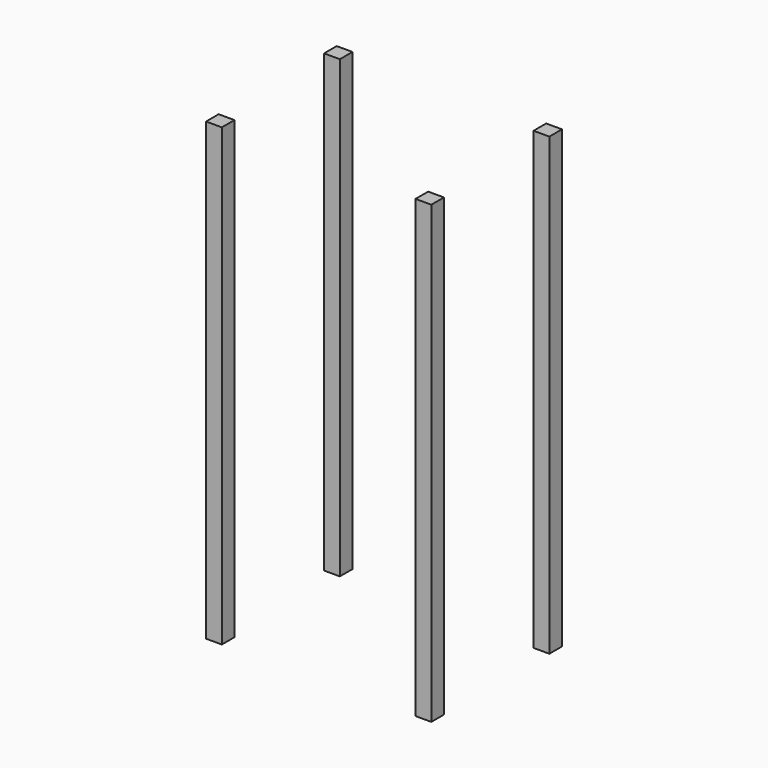
from build123d import *

# Parameters (mm, degrees)
F0_W     = 5.08
F0_H     = 5.08
F1_DEPTH = 146.41856


# Not quite as in the source:
# - the program builds the solid bodies; features that only make, move or delete a surface that nothing else refers to are left out


with BuildPart() as f1:
    # F0 (on Top) → F1 (new body)
    with BuildSketch(Plane.XY):
        with Locations((-33.6806811392, 23.723941824)):
            Rectangle(F0_W, F0_H)
    extrude(amount=F1_DEPTH)


with BuildPart() as f1b:
    # F0 (on Top) → F1, piece 2 (new body)
    with BuildSketch(Plane.XY):
        with Locations((-33.6806811392, -23.723941824)):
            Rectangle(F0_W, F0_H)
    extrude(amount=F1_DEPTH)


with BuildPart() as f1c:
    # F0 (on Top) → F1, piece 3 (new body)
    with BuildSketch(Plane.XY):
        with Locations((33.6806811392, -23.723941824)):
            Rectangle(F0_W, F0_H)
    extrude(amount=F1_DEPTH)


with BuildPart() as f1d:
    # F0 (on Top) → F1, piece 4 (new body)
    with BuildSketch(Plane.XY):
        with Locations((33.6806811392, 23.723941824)):
            Rectangle(F0_W, F0_H)
    extrude(amount=F1_DEPTH)


solid = Compound([f1.part, f1b.part, f1c.part, f1d.part])
